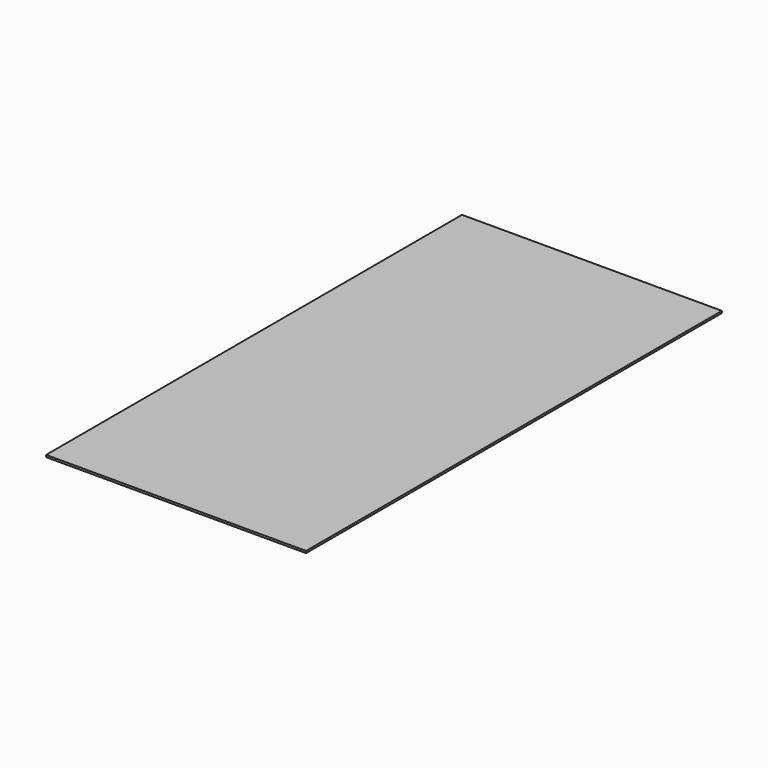
from build123d import *

# Parameters (mm, degrees)
F0_W     = 1219.2
F0_H     = 2438.4
F1_DEPTH = 9.525


# Not quite as in the source:
# - a length typed as a fraction of an inch, garbled in the dataset ("3 / 203.2 mm" for 3/8 in), is restored


with BuildPart() as f1:
    # F0 (on Top) → F1 (new body)
    with BuildSketch(Plane.XY):
        with Locations((-650.8001498044, 1074.5505390882)):
            Rectangle(F0_W, F0_H)
    extrude(amount=F1_DEPTH)


solid = f1.part
